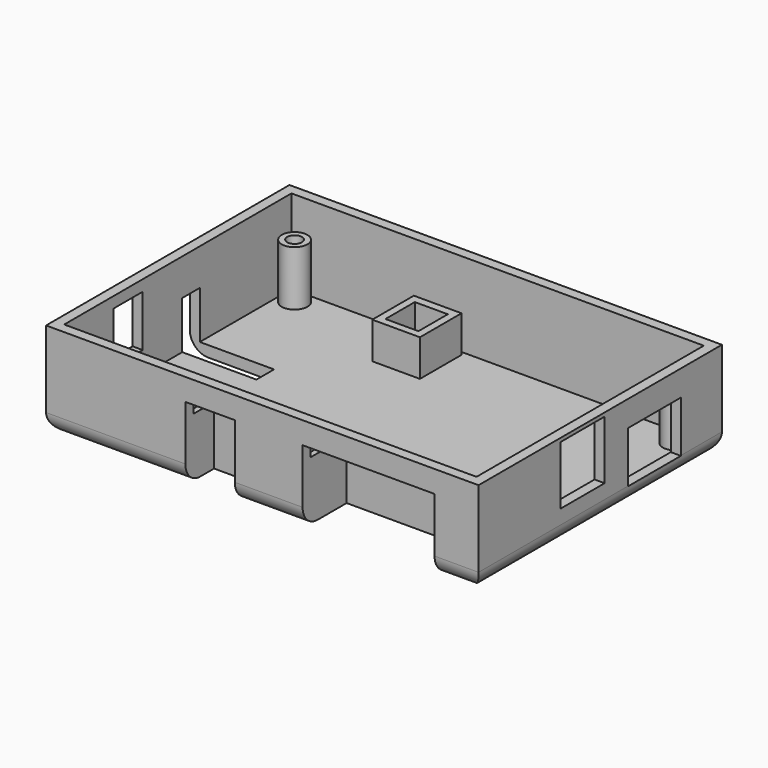
from build123d import *

# Parameters (mm, degrees)
F0_W          = 118
F0_H          = 83
F1_DEPTH      = 26
F2_W          = 112.5
F2_H          = 77.5
F3_DEPTH      = 23
F4_W          = 36
F4_H          = 15
F4_W_2        = 13.5
F4_H_2        = 9.8
F5_DEPTH      = 20
F6_W          = 36
F6_H          = 1.75
F6_W_2        = 13.5
F6_H_2        = 0.95
F7_DEPTH      = 13
F8_W          = 10
F8_H          = 14
F9_DEPTH      = 10
F10_W         = 23
F10_H         = 6
F11_DEPTH     = 16
F12_W         = 9
F12_H         = 10
F13_DEPTH     = 10
F14_W         = 18
F14_H         = 14
F14_W_2       = 15
F14_H_2       = 16
F15_DEPTH     = 10
F16_W         = 9
F16_H         = 2.1789309084
F17_DEPTH     = 10
F18_R         = 3
F19_DEPTH     = 25.4
F20_R         = 3.5
F23_DEPTH     = 15
F21_R         = 3
F24_DEPTH     = 14.7
F22_R         = 2
F25_DEPTH     = 25.4
F26_TEXT_SIZE = 24.7283657599
F27_DEPTH     = 2.54
F28_T1_DEPTH  = 63.4
F28_T3_DEPTH  = 43.9
F28_T5_DEPTH  = 37.4
F28_T7_DEPTH  = 108.4
F28_T9_DEPTH  = 143.4
F28_T11_DEPTH = 59.4
F28_T13_DEPTH = 68.4


# Not quite as in the source:
# - a fillet or chamfer that OpenCascade refuses, or shapes differently, is made with other operations: its cross-section is extruded or revolved along the edge and cut away or added
# - Text() gives the source's letters only with a copy of the font that has no kerning and outlines rounded to 1/6400 em; it was checked with that copy


with BuildPart() as f1:
    # F0 (on Top) → F1 (new body)
    with BuildSketch(Plane.XY):
        Rectangle(F0_W, F0_H)
    extrude(amount=F1_DEPTH)

    # F2 (on face) → F3 (cut)
    with BuildSketch(Plane.XY.offset(26)):
        Rectangle(F2_W, F2_H)
    extrude(amount=-F3_DEPTH, mode=Mode.SUBTRACT)

    # F4 (on face) → F5 (cut)
    with BuildSketch(Plane(origin=(0, 0, 0), x_dir=(1, 0, 0), z_dir=(0, 0, -1))):
        with Locations((29, 34)):
            Rectangle(F4_W, F4_H)
        with Locations((-14.25, 36.6)):
            Rectangle(F4_W_2, F4_H_2)
    extrude(amount=-F5_DEPTH, mode=Mode.SUBTRACT)

    # F6 (on face) → F7 (join)
    with BuildSketch(Plane.XY.offset(3)):
        Polygon((47, -26.5), (47, -38.75), (48, -38.75), (48, -24.75), (47, -24.75), align=None)
        with Locations((29, -25.625)):
            Rectangle(F6_W, F6_H)
        Polygon((11, -38.75), (11, -26.5), (11, -24.75), (9.5, -24.75), (9.5, -38.75), align=None)
        Polygon((-7.5, -31.7), (-7.5, -38.75), (-6.2, -38.75), (-6.2, -30.75), (-7.5, -30.75), align=None)
        with Locations((-14.25, -31.225)):
            Rectangle(F6_W_2, F6_H_2)
        Polygon((-21, -38.75), (-21, -31.7), (-21, -30.75), (-22.5, -30.75), (-22.5, -38.75), align=None)
    extrude(amount=F7_DEPTH)

    # F8 (on face) → F9 (cut)
    with BuildSketch(Plane(origin=(-59, 0, 0), x_dir=(0, -1, 0), z_dir=(-1, 0, 0))):
        with Locations((17, 16)):
            Rectangle(F8_W, F8_H)
    extrude(amount=-F9_DEPTH, mode=Mode.SUBTRACT)

    # F10 (on face) → F11 (cut)
    with BuildSketch(Plane(origin=(0, 0, 0), x_dir=(1, 0, 0), z_dir=(0, 0, -1))):
        with Locations((-47.5, -4.5)):
            Rectangle(F10_W, F10_H)
    extrude(amount=-F11_DEPTH, mode=Mode.SUBTRACT)

    # F12 (on face) → F13 (cut)
    with BuildSketch(Plane(origin=(0, 0, 0), x_dir=(1, 0, 0), z_dir=(0, 0, -1))):
        with Locations((-15.5, -30.5)):
            Rectangle(F12_W, F12_H)
    extrude(amount=-F13_DEPTH, mode=Mode.SUBTRACT)

    # F14 (on face) → F15 (cut)
    with BuildSketch(Plane.YZ.offset(59)):
        with Locations((18.5, 12)):
            Rectangle(F14_W, F14_H)
        with Locations((-6, 17)):
            Rectangle(F14_W_2, F14_H_2)
    extrude(amount=-F15_DEPTH, mode=Mode.SUBTRACT)

    # F16 (on face) → F17 (join)
    with BuildSketch(Plane.XY.offset(3)):
        Polygon((-22, 37.6789309084), (-22, 25.5), (-20, 25.5), (-20, 35.5), (-20, 37.6789309084), align=None)
        Polygon((-20, 25.5), (-22, 25.5), (-22, 23.5), (-11, 23.5), (-11, 25.5), align=None)
        Polygon((-11, 35.5), (-11, 25.5), (-11, 23.5), (-9, 23.5), (-9, 37.6789309084), (-11, 37.6789309084), align=None)
        with Locations((-15.5, 36.5894654542)):
            Rectangle(F16_W, F16_H)
    extrude(amount=F17_DEPTH)

    # F18 (on face) → F19 (cut)
    with BuildSketch(Plane(origin=(0, 0, 0), x_dir=(1, 0, 0), z_dir=(0, 0, -1))):
        with Locations((-52, -34.5)):
            Circle(F18_R)
        with Locations((-52, 34.5)):
            Circle(F18_R)
        with Locations((52, -34.5)):
            Circle(F18_R)
        with Locations((52, 34.5)):
            Circle(F18_R)
    extrude(amount=-F19_DEPTH, mode=Mode.SUBTRACT)

    # F20 (on face) → F23 (join)
    with BuildSketch(Plane.XY.offset(3)):
        with Locations((-52, 34.5)):
            Circle(F20_R)
        with Locations((-52, -34.5)):
            Circle(F20_R)
        with Locations((52, -34.5)):
            Circle(F20_R)
        with Locations((52, 34.5)):
            Circle(F20_R)
    extrude(amount=F23_DEPTH)

    # F21 (on face) → F24 (cut)
    with BuildSketch(Plane(origin=(0, 0, 0), x_dir=(1, 0, 0), z_dir=(0, 0, -1))):
        with Locations((52, -34.5)):
            Circle(F21_R)
        with Locations((-52, -34.5)):
            Circle(F21_R)
        with Locations((52, 34.5)):
            Circle(F21_R)
        with Locations((-52, 34.5)):
            Circle(F21_R)
    extrude(amount=-F24_DEPTH, mode=Mode.SUBTRACT)

    # F22 (on face) → F25 (cut)
    with BuildSketch(Plane(origin=(0, 0, 0), x_dir=(1, 0, 0), z_dir=(0, 0, -1))):
        with Locations((-52, 34.5)):
            Circle(F22_R)
        with Locations((52, 34.5)):
            Circle(F22_R)
        with Locations((52, -34.5)):
            Circle(F22_R)
        with Locations((-52, -34.5)):
            Circle(F22_R)
    extrude(amount=-F25_DEPTH, mode=Mode.SUBTRACT)

    # F26 (on face) → F27 (cut)
    with BuildSketch(Plane(origin=(0, 0, 0), x_dir=(1, 0, 0), z_dir=(0, 0, -1))):
        with Locations((-33.472660929, -8.4710698575)):
            Text('Dong-A', F26_TEXT_SIZE, font='Open Sans', text_align=(TextAlign.LEFT, TextAlign.BOTTOM))
    extrude(amount=-F27_DEPTH, mode=Mode.SUBTRACT)

    # F28: fillet of radius 5.08 on 7 edges, made by hand

    # F28_s2 → F28_t1 (cut)
    with BuildSketch(Plane.YZ.offset(-71.7)):
        with BuildLine():
            ThreePointArc((-41.5, 5.08), (-40.0121024484, 1.4878975516), (-36.42, 0))
            Line((-36.42, 0), (-41.5, 0))
            Line((-41.5, 0), (-41.5, 5.08))
        make_face()
    extrude(amount=F28_T1_DEPTH, mode=Mode.SUBTRACT)

    # F28_s4 → F28_t3 (cut)
    with BuildSketch(Plane.YZ.offset(-20.2)):
        with BuildLine():
            ThreePointArc((-41.5, 5.08), (-40.0121024484, 1.4878975516), (-36.42, 0))
            Line((-36.42, 0), (-41.5, 0))
            Line((-41.5, 0), (-41.5, 5.08))
        make_face()
    extrude(amount=F28_T3_DEPTH, mode=Mode.SUBTRACT)

    # F28_s6 → F28_t5 (cut)
    with BuildSketch(Plane.YZ.offset(34.3)):
        with BuildLine():
            ThreePointArc((-41.5, 5.08), (-40.0121024484, 1.4878975516), (-36.42, 0))
            Line((-36.42, 0), (-41.5, 0))
            Line((-41.5, 0), (-41.5, 5.08))
        make_face()
    extrude(amount=F28_T5_DEPTH, mode=Mode.SUBTRACT)

    # F28_s8 → F28_t7 (cut)
    with BuildSketch(Plane.XZ.offset(-54.2)):
        with BuildLine():
            ThreePointArc((53.92, 0), (57.5121024484, 1.4878975516), (59, 5.08))
            Line((59, 5.08), (59, 0))
            Line((59, 0), (53.92, 0))
        make_face()
    extrude(amount=F28_T7_DEPTH, mode=Mode.SUBTRACT)

    # F28_s10 → F28_t9 (cut)
    with BuildSketch(Plane.YZ.offset(-71.7)):
        with BuildLine():
            ThreePointArc((36.42, 0), (40.0121024484, 1.4878975516), (41.5, 5.08))
            Line((41.5, 5.08), (41.5, 0))
            Line((41.5, 0), (36.42, 0))
        make_face()
    extrude(amount=F28_T9_DEPTH, mode=Mode.SUBTRACT)

    # F28_s12 → F28_t11 (cut)
    with BuildSketch(Plane.XZ.offset(-54.2)):
        with BuildLine():
            ThreePointArc((-53.92, 0), (-57.5121024484, 1.4878975516), (-59, 5.08))
            Line((-59, 5.08), (-59, 0))
            Line((-59, 0), (-53.92, 0))
        make_face()
    extrude(amount=F28_T11_DEPTH, mode=Mode.SUBTRACT)

    # F28_s14 → F28_t13 (cut)
    with BuildSketch(Plane.XZ.offset(-14.2)):
        with BuildLine():
            ThreePointArc((-53.92, 0), (-57.5121024484, 1.4878975516), (-59, 5.08))
            Line((-59, 5.08), (-59, 0))
            Line((-59, 0), (-53.92, 0))
        make_face()
    extrude(amount=F28_T13_DEPTH, mode=Mode.SUBTRACT)


solid = f1.part
